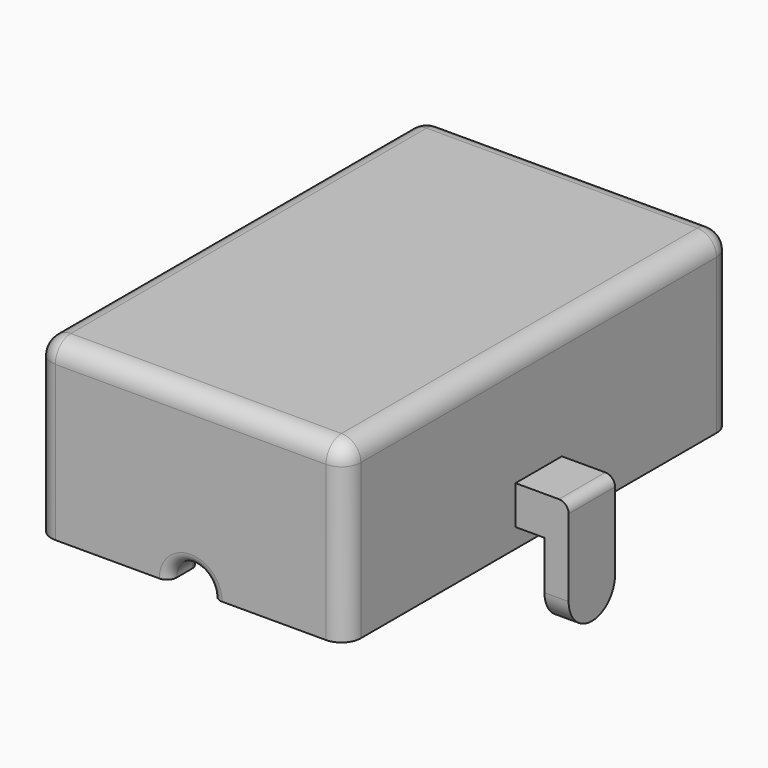
from build123d import *

# Parameters (mm, degrees)
F0_W      = 16
F0_H      = 25
F1_DEPTH  = 9
F2_T      = -2
F5_DEPTH  = 2
F6_R      = 1.25
F7_DEPTH  = 12
F8_R      = 1
F9_R      = 1.125
F10_DEPTH = 12.5
F12_DEPTH = 1.5
F14_DEPTH = 5
F15_R     = 0.5
F16_R     = 0.49999


# Not quite as in the source:
# - a fillet or chamfer is up to 0.001 mm smaller than in the source, because OpenCascade refuses the exact size


with BuildPart() as f1:
    # F0 (on Top) → F1 (new body)
    with BuildSketch(Plane.XY):
        Rectangle(F0_W, F0_H)
    extrude(amount=-F1_DEPTH)

    # F2
    f2_openings = [f1.faces().sort_by_distance(p)[0] for p in [
        (0, 0, -9),
    ]]
    offset(amount=F2_T, openings=f2_openings)

    # F4 (on offset) → F5 (join)
    with BuildSketch(Plane(origin=(0, 8.25, 0), x_dir=(-1, 0, 0), z_dir=(0, 1, 0))):
        with BuildLine():
            Line((8, -9), (11.375, -9))
            ThreePointArc((11.375, -9), (13.1043679152, -6.9820697596), (10.8454571871, -5.5820418442))
            ThreePointArc((10.8454571871, -5.5820418442), (8.8945109421, -5.2629183791), (8, -3.5))
            Line((8, -3.5), (8, -9))
        make_face()
    extrude(amount=-F5_DEPTH)

    # F6 (on face) → F7 (join)
    with BuildSketch(Plane.XZ.offset(-6.25)):
        with Locations((-11.375, -7.25)):
            Circle(F6_R)
    extrude(amount=F7_DEPTH)

    # F8
    f8_edges = [f1.edges().sort_by_distance(p)[0] for p in [
        (0, 12.5, 0),
        (-8, 12.5, -4.5),
        (-8, 0, 0),
        (-8, -12.5, -4.5),
        (8, 0, 0),
        (8, 12.5, -4.5),
        (8, -12.5, -4.5),
        (0, -12.5, 0),
    ]]
    fillet(f8_edges, radius=F8_R)

    # F9 (on Front) → F10 (cut, symmetric)
    with BuildSketch(Plane.XZ):
        with Locations((0, -9)):
            Circle(F9_R)
    extrude(amount=F10_DEPTH, both=True, mode=Mode.SUBTRACT)

    # F11 (on Front) → F12 (join, symmetric)
    with BuildSketch(Plane.XZ):
        Polygon((10.75, -12), (10.75, -6), (8, -6), (8, -8), (9.5, -8), (9.5, -12), align=None)
    extrude(amount=F12_DEPTH, both=True)

    # F13 (on face) → F14 (cut)
    with BuildSketch(Plane.YZ.offset(10.75)):
        with BuildLine():
            ThreePointArc((1.5, -10.5), (1.0606601718, -11.5606601718), (0, -12))
            Line((0, -12), (1.5, -12))
            Line((1.5, -12), (1.5, -10.5))
        make_face()
        with BuildLine():
            ThreePointArc((0, -12), (-1.0606601718, -11.5606601718), (-1.5, -10.5))
            Line((-1.5, -10.5), (-1.5, -12))
            Line((-1.5, -12), (0, -12))
        make_face()
    extrude(amount=-F14_DEPTH, mode=Mode.SUBTRACT)

    # F15
    f15_edges = [f1.edges().sort_by_distance(p)[0] for p in [
        (10.75, 0, -6),
    ]]
    fillet(f15_edges, radius=F15_R)

    # F16 (radius 0.5 in the source; OpenCascade refuses exactly that, so slightly less here)
    f16_edges = [f1.edges().sort_by_distance(p)[0] for p in [
        (-12.625, 6.25, -7.25),
        (0, -12.5, -7.875),
        (0, -10.5, -7.875),
        (0, 12.5, -7.875),
        (0, 10.5, -7.875),
    ]]
    fillet(f16_edges, radius=F16_R)


solid = f1.part
